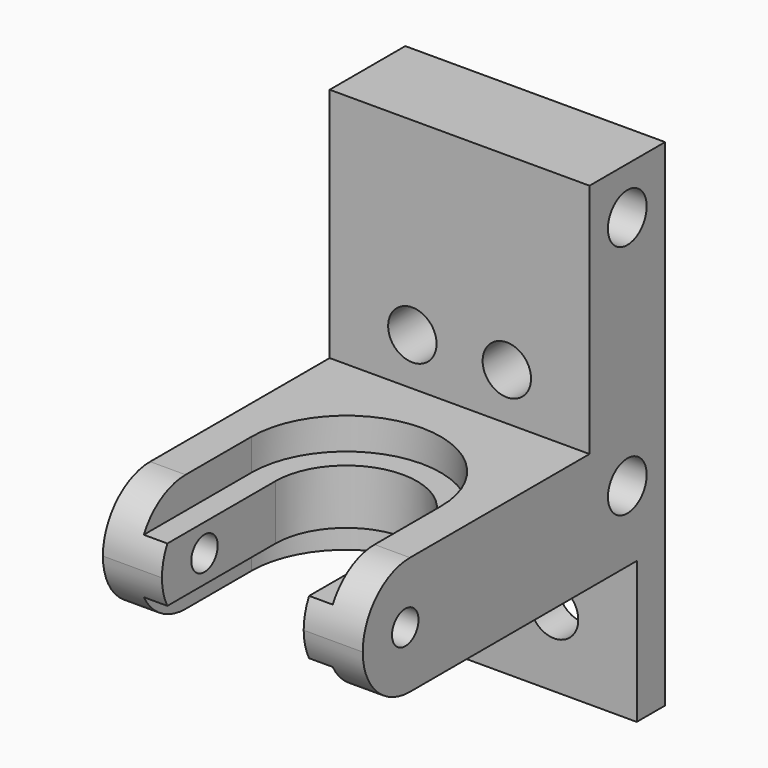
from build123d import *

# Parameters (mm, degrees)
F0_W     = 22
F0_H     = 42
F1_DEPTH = 3
F2_W     = 3
F2_H     = 30
F2_W_2   = 5
F3_DEPTH = 22
F4_D     = 4.1
F7_DEPTH = 5
F8_DEPTH = 2.325
F9_R     = 4.99999
F11_D    = 4.1
F12_D    = 2.8


# Not quite as in the source:
# - a fillet or chamfer is up to 0.001 mm smaller than in the source, because OpenCascade refuses the exact size


with BuildPart() as f1:
    # F0 (on Front) → F1 (new body)
    with BuildSketch(Plane.XZ):
        with Locations((-28.9233987555, 27.9422005266)):
            Rectangle(F0_W, F0_H)
    extrude(amount=F1_DEPTH)

    # F2 (on face) → F3 (join)
    with BuildSketch(Plane(origin=(-39.9233987555, 0, 0), x_dir=(0, -1, 0), z_dir=(-1, 0, 0))):
        with Locations((1.5, 33.9422005266)):
            Rectangle(F2_W, F2_H)
        with Locations((5.5, 33.9422005266)):
            Rectangle(F2_W_2, F2_H)
    extrude(amount=-F3_DEPTH)

    # F4 (through all)
    with Locations(Plane(origin=(0, 0, 0), x_dir=(1, 0, 0), z_dir=(0, 1, 0))):
        with Locations((-24.9233987555, -12.9422005266), (-32.9233987555, -12.9422005266), (-32.9233987555, -32.9422005266), (-24.9233987555, -32.9422005266)):
            Hole(F4_D / 2)

    # F6 (on line) → F7 (join, symmetric)
    with BuildSketch(Plane.XY.offset(23.9422005266)):
        with BuildLine():
            ThreePointArc((-36.9233987555, -20), (-28.9233987555, -12), (-20.9233987555, -20))
            Line((-20.9233987555, -20), (-20.9233987555, -32))
            Line((-20.9233987555, -32), (-17.9233987555, -32))
            Line((-17.9233987555, -32), (-17.9233987555, 0))
            Line((-17.9233987555, 0), (-39.9233987555, 0))
            Line((-39.9233987555, 0), (-39.9233987555, -32))
            Line((-39.9233987555, -32), (-36.9233987555, -32))
            Line((-36.9233987555, -32), (-36.9233987555, -20))
        make_face()
    extrude(amount=F7_DEPTH, both=True)

    # F6 (on line) → F8 (join, symmetric)
    with BuildSketch(Plane.XY.offset(23.9422005266)):
        with BuildLine():
            ThreePointArc((-34.9233987555, -20), (-28.9233987555, -14), (-22.9233987555, -20))
            Line((-22.9233987555, -20), (-22.9233987555, -25.2915026221))
            ThreePointArc((-22.9233987555, -25.2915026221), (-21.4400839819, -22.8284271247), (-20.9233987555, -20))
            ThreePointArc((-20.9233987555, -20), (-28.9233987555, -12), (-36.9233987555, -20))
            ThreePointArc((-36.9233987555, -20), (-36.406713529, -22.8284271247), (-34.9233987555, -25.2915026221))
            Line((-34.9233987555, -25.2915026221), (-34.9233987555, -20))
        make_face()
        with BuildLine():
            Line((-34.9233987555, -32), (-34.9233987555, -25.2915026221))
            ThreePointArc((-34.9233987555, -25.2915026221), (-36.406713529, -22.8284271247), (-36.9233987555, -20))
            Line((-36.9233987555, -20), (-36.9233987555, -32))
            Line((-36.9233987555, -32), (-34.9233987555, -32))
        make_face()
        with BuildLine():
            ThreePointArc((-20.9233987555, -20), (-21.4400839819, -22.8284271247), (-22.9233987555, -25.2915026221))
            Line((-22.9233987555, -25.2915026221), (-22.9233987555, -32))
            Line((-22.9233987555, -32), (-20.9233987555, -32))
            Line((-20.9233987555, -32), (-20.9233987555, -20))
        make_face()
    extrude(amount=F8_DEPTH, both=True)

    # F9 (radius 5 in the source; OpenCascade refuses exactly that, so slightly less here)
    f9_edges = [f1.edges().sort_by_distance(p)[0] for p in [
        (-38.423399, -32, 28.942201),
        (-38.423399, -32, 18.942201),
        (-19.423399, -32, 18.942201),
        (-19.423399, -32, 28.942201),
    ]]
    fillet(f9_edges, radius=F9_R)

    # F11 (through all)
    with Locations(Plane(origin=(-39.9233987555, 0, 0), x_dir=(0, -1, 0), z_dir=(-1, 0, 0))):
        with Locations((4, 44.9422005266), (4, 24.9422005266)):
            Hole(F11_D / 2)

    # F12 (through all)
    with Locations(Plane(origin=(-39.9233987555, 0, 0), x_dir=(0, -1, 0), z_dir=(-1, 0, 0))):
        with Locations((27.5, 23.9422005266)):
            Hole(F12_D / 2)


solid = f1.part
